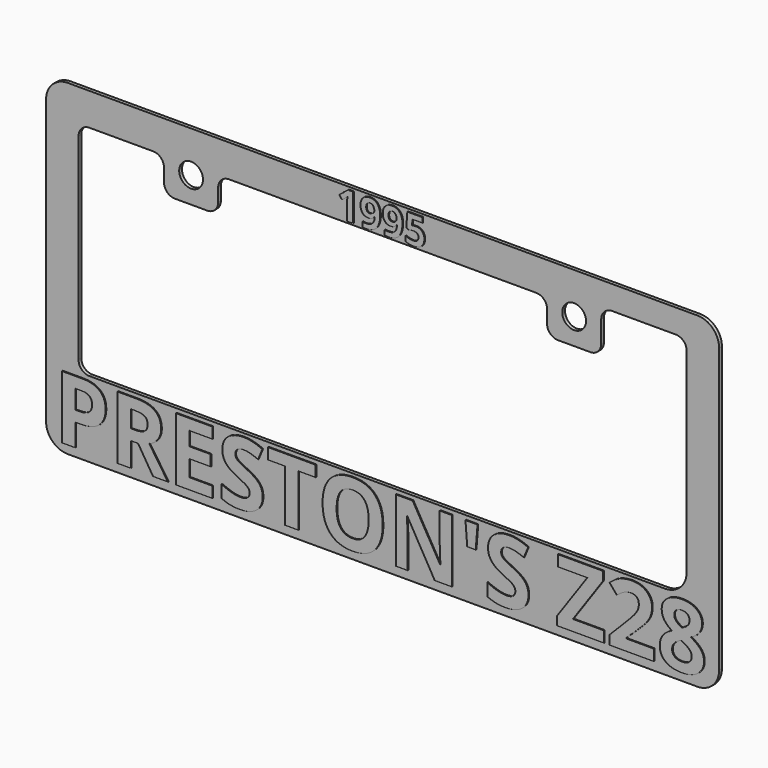
from build123d import *

# Parameters (mm, degrees)
F1_DEPTH      = 1.6
F2_W          = 25
F2_H          = 16
F3_DEPTH      = 1.6
F5_DEPTH      = 25
F6_R          = 5
F8_R          = 5.5
F9_DEPTH      = 25
F10_TEXT_SIZE = 18.0555555556
F11_DEPTH     = 0.4
F12_TEXT_SIZE = 40.8665598921
F13_DEPTH     = 0.4


# Not quite as in the source:
# - two fillets or chamfers of one size are made in one step
# - Text() gives the source's letters only with a copy of the font that has no kerning and outlines rounded to 1/6400 em; it was checked with that copy


with BuildPart() as f1:
    # F0 (on Front) → F1 (new body)
    with BuildSketch(Plane.XZ):
        with BuildLine():
            ThreePointArc((155.5, 65.5), (152.5710678119, 72.5710678119), (145.5, 75.5))
            Line((145.5, 75.5), (-145.5, 75.5))
            ThreePointArc((-145.5, 75.5), (-152.5710678119, 72.5710678119), (-155.5, 65.5))
            Line((-155.5, 65.5), (-155.5, -65.5))
            ThreePointArc((-155.5, -65.5), (-152.5710678119, -72.5710678119), (-145.5, -75.5))
            Line((-145.5, -75.5), (145.5, -75.5))
            ThreePointArc((145.5, -75.5), (152.5710678119, -72.5710678119), (155.5, -65.5))
            Line((155.5, -65.5), (155.5, 65.5))
        make_face()
        with BuildLine():
            Line((-135.5, 60.5), (135.5, 60.5))
            ThreePointArc((135.5, 60.5), (139.0355339059, 59.0355339059), (140.5, 55.5))
            Line((140.5, 55.5), (140.5, -30.5))
            ThreePointArc((140.5, -30.5), (137.5710678119, -37.5710678119), (130.5, -40.5))
            Line((130.5, -40.5), (-135.5, -40.5))
            ThreePointArc((-135.5, -40.5), (-139.0355339059, -39.0355339059), (-140.5, -35.5))
            Line((-140.5, -35.5), (-140.5, 55.5))
            ThreePointArc((-140.5, 55.5), (-139.0355339059, 59.0355339059), (-135.5, 60.5))
        make_face(mode=Mode.SUBTRACT)
    extrude(amount=F1_DEPTH)

    # F2 (on face) → F3 (join, through all)
    with BuildSketch(Plane.XZ.offset(1.6)):
        with Locations((-88.5, 52.5)):
            Rectangle(F2_W, F2_H)
        with Locations((88.5, 52.5)):
            Rectangle(F2_W, F2_H)
    extrude(amount=-F3_DEPTH)

    # F4 (on face) → F5 (cut)
    with BuildSketch(Plane.XZ.offset(1.6)):
        Polygon((101, 64.5), (101, 60.5), (101, 55.5), (140.5, 55.5), (140.5, 64.5), align=None)
    extrude(amount=-F5_DEPTH, mode=Mode.SUBTRACT)

    # F6
    f6_edges = [f1.edges().sort_by_distance(p)[0] for p in [
        (-101, -0.8, 44.5),
        (-101, -0.8, 60.5),
        (-76, -0.8, 44.5),
        (-76, -0.8, 60.5),
        (101, -0.8, 44.5),
        (76, -0.8, 44.5),
        (76, -0.8, 60.5),
        (140.5, -0.8, 64.5),
        (101, -0.8, 64.5),
    ]]
    fillet(f6_edges, radius=F6_R)

    # F8 (on face) → F9 (cut)
    with BuildSketch(Plane.XZ.offset(1.6)):
        with Locations((-88.5, 56.5)):
            Circle(F8_R)
        with Locations((88.5, 56.5)):
            Circle(F8_R)
    extrude(amount=-F9_DEPTH, mode=Mode.SUBTRACT)

    # F10 (on face) → F11 (join)
    with BuildSketch(Plane.XZ.offset(1.6)):
        with Locations((-20.7921006944, 61.5)):
            Text('1995', F10_TEXT_SIZE, font='Open Sans', font_style=FontStyle.BOLD, text_align=(TextAlign.LEFT, TextAlign.BOTTOM))
    extrude(amount=F11_DEPTH)

    # F12 (on face) → F13 (join)
    with BuildSketch(Plane.XZ.offset(1.6)):
        with Locations((-151.5, -71.5)):
            Text("PRESTON'S Z28", F12_TEXT_SIZE, font='Open Sans', font_style=FontStyle.BOLD, text_align=(TextAlign.LEFT, TextAlign.BOTTOM))
    extrude(amount=F13_DEPTH)


solid = f1.part
